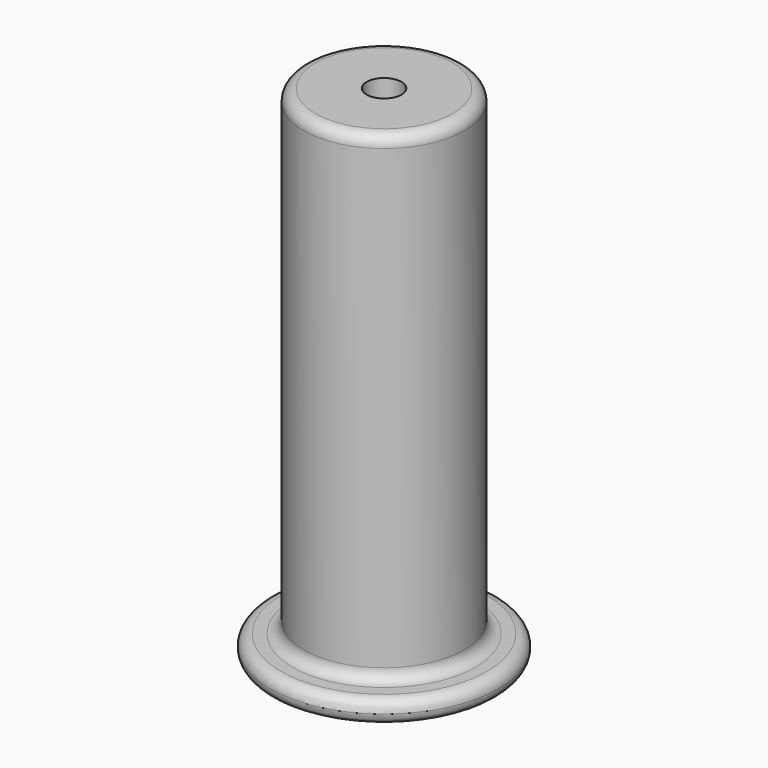
from build123d import *

# Parameters (mm, degrees)
F0_R     = 25
F1_DEPTH = 5
F2_R     = 17.5
F3_DEPTH = 105
F4_R     = 15.5
F5_DEPTH = 105
F6_R     = 2.49999
F7_R     = 3.8034251557
F8_DEPTH = 30


# Not quite as in the source:
# - a fillet or chamfer is up to 0.001 mm smaller than in the source, because OpenCascade refuses the exact size


with BuildPart() as f1:
    # F0 (on Top) → F1 (new body)
    with BuildSketch(Plane.XY):
        Circle(F0_R)
    extrude(amount=F1_DEPTH)

    # F2 (on face) → F3 (join)
    with BuildSketch(Plane.XY.offset(5)):
        Circle(F2_R)
    extrude(amount=F3_DEPTH)

    # F4 (on face) → F5 (cut)
    with BuildSketch(Plane(origin=(0, 0, 0), x_dir=(1, 0, 0), z_dir=(0, 0, -1))):
        Circle(F4_R)
    extrude(amount=-F5_DEPTH, mode=Mode.SUBTRACT)

    # F6 (radius 2.5 in the source; OpenCascade refuses exactly that, so slightly less here)
    f6_edges = [f1.edges().sort_by_distance(p)[0] for p in [
        (-17.5, 0, 110),
        (-17.5, 0, 5),
        (-25, 0, 5),
        (-25, 0, 0),
    ]]
    fillet(f6_edges, radius=F6_R)

    # F7 (on face) → F8 (cut)
    with BuildSketch(Plane.XY.offset(110)):
        Circle(F7_R)
    extrude(amount=-F8_DEPTH, mode=Mode.SUBTRACT)


solid = f1.part
